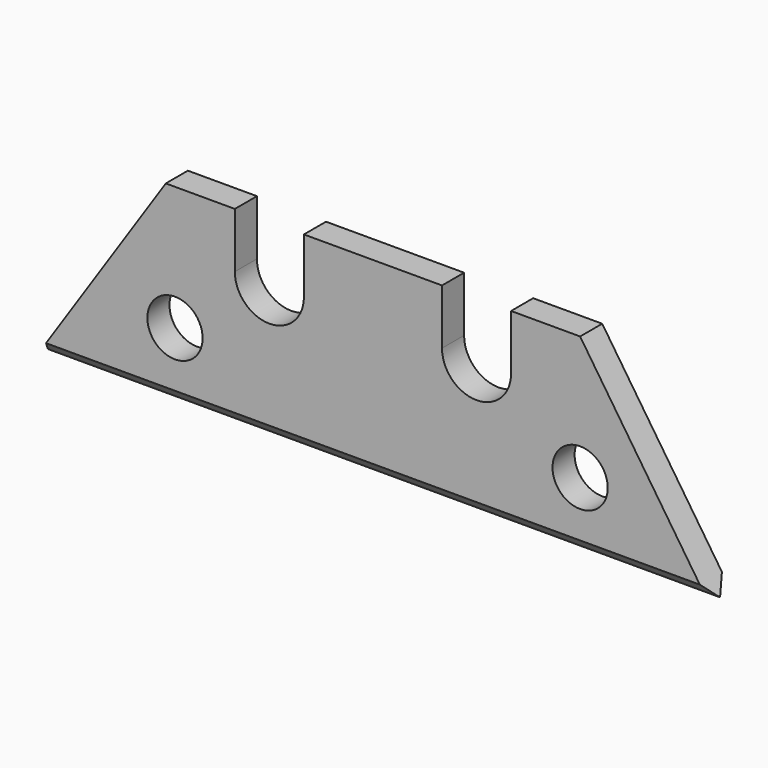
from build123d import *

# Parameters (mm, degrees)
F1_DEPTH    = 2.54
F2_T1_DEPTH = 76.5641495789
F3_R        = 2.54
F4_DEPTH    = 2.54


# Not quite as in the source:
# - a fillet or chamfer that OpenCascade refuses, or shapes differently, is made with other operations: its cross-section is extruded or revolved along the edge and cut away or added


with BuildPart() as f1:
    # F0 (on Front) → F1 (new body)
    with BuildSketch(Plane.XZ):
        with BuildLine():
            Line((-63.5, 0), (0, 0))
            Line((0, 0), (-12.7, 19.05))
            Line((-12.7, 19.05), (-19.05, 19.05))
            Line((-19.05, 19.05), (-19.05, 13.97))
            ThreePointArc((-19.05, 13.97), (-22.225, 10.795), (-25.4, 13.97))
            Line((-25.4, 13.97), (-25.4, 19.05))
            Line((-25.4, 19.05), (-38.1, 19.05))
            Line((-38.1, 19.05), (-38.1, 13.97))
            ThreePointArc((-38.1, 13.97), (-41.275, 10.795), (-44.45, 13.97))
            Line((-44.45, 13.97), (-44.45, 19.05))
            Line((-44.45, 19.05), (-50.8, 19.05))
            Line((-50.8, 19.05), (-63.5, 0))
        make_face()
    extrude(amount=F1_DEPTH)

    # F2: chamfer of 2.54 on 2 edges, made by hand

    # F2_s2 → F2_t1 (cut)
    with BuildSketch(Plane.YZ.offset(-70.0320747894)):
        Polygon((0, 0), (-2.54, 2.54), (-2.54, 0), align=None)
        Polygon((-2.54, 0), (0, 2.54), (0, 0), align=None)
    extrude(amount=F2_T1_DEPTH, mode=Mode.SUBTRACT)

    # F3 (on face) → F4 (cut)
    with BuildSketch(Plane.XZ.offset(2.54)):
        with Locations((-12.7, 7.62)):
            Circle(F3_R)
        with Locations((-49.9533333333, 7.62)):
            Circle(F3_R)
    extrude(amount=-F4_DEPTH, mode=Mode.SUBTRACT)


solid = f1.part
